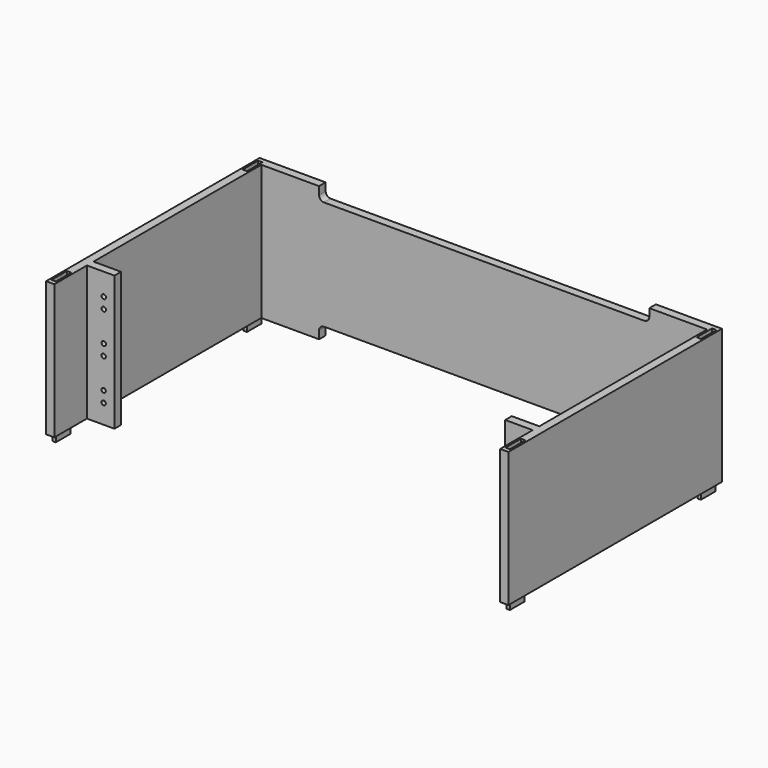
from build123d import *

# Parameters (mm, degrees)
F0_W          = 5
F0_H          = 1.5
F0_W_2        = 0.8
F0_H_2        = 3.5
F0_W_3        = 0.6
F0_H_3        = 3.3
F0_H_4        = 2.7
F0_H_5        = 0.6
F1_DEPTH      = 23
F1_DEPTH_BACK = 1.5
F3_D          = 0.8
F3_DEPTH      = 2
F3_TIP        = 0.2403442476
F5_D          = 0.8
F5_DEPTH      = 2
F5_TIP        = 0.2403442476
F6_DEPTH      = 2.8
F7_START      = 21.5
F7_DEPTH      = 1.5
F9_DEPTH      = 2


# Not quite as in the source:
# - a feature names something its author has since deleted; it is built from what else it names


with BuildPart() as f1:
    # F0 (on Top) → F1 (new body, two sides)
    with BuildSketch(Plane.XY) as f1_sk:
        with Locations((-38.0453250408, -14.9690947816)):
            Rectangle(F0_W, F0_H)
        Polygon((-42.0453250408, -23.1190947816), (-40.5453250408, -23.1190947816), (-40.5453250408, -15.7190947816), (-40.5453250408, -14.2190947816), (-40.5453250408, 23.8809052184), (-40.8953250408, 23.8809052184), (-40.8953250408, 21.0809052184), (-41.6953250408, 21.0809052184), (-41.6953250408, 23.8809052184), (-42.0453250408, 23.8809052184), align=None)
        with Locations((-41.2953250408, -20.5690947816)):
            Rectangle(F0_W_2, F0_H_2, mode=Mode.SUBTRACT)
        Polygon((-42.0453250408, 25.3809052184), (-42.0453250408, 23.8809052184), (-41.6953250408, 23.8809052184), (-41.6953250408, 24.5809052184), (-40.8953250408, 24.5809052184), (-40.8953250408, 23.8809052184), (-40.5453250408, 23.8809052184), (40.4546749592, 23.8809052184), (40.8046749592, 23.8809052184), (40.8046749592, 24.5809052184), (41.6046749592, 24.5809052184), (41.6046749592, 23.8809052184), (41.9546749592, 23.8809052184), (41.9546749592, 25.3809052184), align=None)
        Polygon((40.8046749592, 23.8809052184), (40.4546749592, 23.8809052184), (40.4546749592, -14.2186603174), (40.4546749592, -15.7186603174), (40.4546749592, -23.1190947816), (41.9546749592, -23.1190947816), (41.9546749592, 23.8809052184), (41.6046749592, 23.8809052184), (41.6046749592, 21.0809052184), (40.8046749592, 21.0809052184), align=None)
        with Locations((41.2046749592, -20.5690947816)):
            Rectangle(F0_W_2, F0_H_2, mode=Mode.SUBTRACT)
        with Locations((37.9546749592, -14.9686603174)):
            Rectangle(F0_W, F0_H)
        with Locations((-41.2953250408, -20.5690947816)):
            Rectangle(F0_W_2, F0_H_2)
        with Locations((-41.2953250408, -20.5690947816)):
            Rectangle(F0_W_3, F0_H_3, mode=Mode.SUBTRACT)
        with Locations((41.2046749592, -20.5690947816)):
            Rectangle(F0_W_2, F0_H_2)
        with Locations((41.2046749592, -20.5690947816)):
            Rectangle(F0_W_3, F0_H_3, mode=Mode.SUBTRACT)
        Polygon((40.9046749592, 23.8809052184), (40.8046749592, 23.8809052184), (40.8046749592, 21.0809052184), (41.6046749592, 21.0809052184), (41.6046749592, 23.8809052184), (41.5046749592, 23.8809052184), (41.5046749592, 21.1809052184), (40.9046749592, 21.1809052184), align=None)
        Polygon((40.8046749592, 24.5809052184), (40.8046749592, 23.8809052184), (40.9046749592, 23.8809052184), (40.9046749592, 24.4809052184), (41.5046749592, 24.4809052184), (41.5046749592, 23.8809052184), (41.6046749592, 23.8809052184), (41.6046749592, 24.5809052184), align=None)
        Polygon((-41.6953250408, 24.5809052184), (-41.6953250408, 23.8809052184), (-41.5953250408, 23.8809052184), (-41.5953250408, 24.4809052184), (-40.9953250408, 24.4809052184), (-40.9953250408, 23.8809052184), (-40.8953250408, 23.8809052184), (-40.8953250408, 24.5809052184), align=None)
        Polygon((-41.5953250408, 23.8809052184), (-41.6953250408, 23.8809052184), (-41.6953250408, 21.0809052184), (-40.8953250408, 21.0809052184), (-40.8953250408, 23.8809052184), (-40.9953250408, 23.8809052184), (-40.9953250408, 21.1809052184), (-41.5953250408, 21.1809052184), align=None)
        with Locations((-41.2953250408, -20.5690947816)):
            Rectangle(F0_W_3, F0_H_3)
        with Locations((-41.2953250408, 22.5309052184)):
            Rectangle(F0_W_3, F0_H_4)
        with Locations((41.2046749592, -20.5690947816)):
            Rectangle(F0_W_3, F0_H_3)
        with Locations((41.2046749592, 22.5309052184)):
            Rectangle(F0_W_3, F0_H_4)
        with Locations((41.2046749592, 24.1809052184)):
            Rectangle(F0_W_3, F0_H_5)
        with Locations((-41.2953250408, 24.1809052184)):
            Rectangle(F0_W_3, F0_H_5)
    extrude(amount=F1_DEPTH)
    extrude(f1_sk.sketch, amount=-F1_DEPTH_BACK)

    # F3
    with Locations(Plane.XZ.offset(15.7190947816)):
        with Locations((-37.4758429825, 18.9999998622), (-37.4758429825, 16.9999998622), (-37.4758429825, 11.4999998622), (-37.5126936273, 9.5), (-37.5126936273, 3.9999998622), (-37.5126936273, 2)):
            Hole(F3_D / 2, depth=F3_DEPTH)
            with Locations((0, 0, -(F3_DEPTH + F3_TIP / 2))):  # 118° drill point
                Cone(0, F3_D / 2, F3_TIP, mode=Mode.SUBTRACT)

    # F5
    with Locations(Plane.XZ.offset(15.7186603174)):
        with Locations((37.5221328411, 19.00000019), (37.5221328411, 17.00000019), (37.5221328411, 11.50000019), (37.4725908041, 9.5000003278), (37.4725908041, 4.00000019), (37.4725908041, 2.0000003278)):
            Hole(F5_D / 2, depth=F5_DEPTH)
            with Locations((0, 0, -(F5_DEPTH + F5_TIP / 2))):  # 118° drill point
                Cone(0, F5_D / 2, F5_TIP, mode=Mode.SUBTRACT)

    # F0 (on Top) → F6 (join)
    with BuildSketch(Plane.XY):
        with Locations((-41.2953250408, 22.5309052184)):
            Rectangle(F0_W_3, F0_H_4)
        with Locations((-41.2953250408, 24.1809052184)):
            Rectangle(F0_W_3, F0_H_5)
        with Locations((-41.2953250408, -20.5690947816)):
            Rectangle(F0_W_3, F0_H_3)
        with Locations((41.2046749592, 22.5309052184)):
            Rectangle(F0_W_3, F0_H_4)
        with Locations((41.2046749592, 24.1809052184)):
            Rectangle(F0_W_3, F0_H_5)
        with Locations((41.2046749592, -20.5690947816)):
            Rectangle(F0_W_3, F0_H_3)
    extrude(amount=-F6_DEPTH)

    # F0 (on Top) → F7 (cut)
    with BuildSketch(Plane.XY.offset(F7_START)):
        with Locations((-41.2953250408, -20.5690947816)):
            Rectangle(F0_W_2, F0_H_2)
        with Locations((-41.2953250408, -20.5690947816)):
            Rectangle(F0_W_3, F0_H_3, mode=Mode.SUBTRACT)
        with Locations((41.2046749592, -20.5690947816)):
            Rectangle(F0_W_2, F0_H_2)
        with Locations((41.2046749592, -20.5690947816)):
            Rectangle(F0_W_3, F0_H_3, mode=Mode.SUBTRACT)
        with Locations((-41.2953250408, -20.5690947816)):
            Rectangle(F0_W_3, F0_H_3)
        with Locations((41.2046749592, -20.5690947816)):
            Rectangle(F0_W_3, F0_H_3)
        with Locations((-41.2953250408, 22.5309052184)):
            Rectangle(F0_W_3, F0_H_4)
        with Locations((41.2046749592, 22.5309052184)):
            Rectangle(F0_W_3, F0_H_4)
        Polygon((-41.5953250408, 23.8809052184), (-41.6953250408, 23.8809052184), (-41.6953250408, 21.0809052184), (-40.8953250408, 21.0809052184), (-40.8953250408, 23.8809052184), (-40.9953250408, 23.8809052184), (-40.9953250408, 21.1809052184), (-41.5953250408, 21.1809052184), align=None)
        Polygon((40.9046749592, 23.8809052184), (40.8046749592, 23.8809052184), (40.8046749592, 21.0809052184), (41.6046749592, 21.0809052184), (41.6046749592, 23.8809052184), (41.5046749592, 23.8809052184), (41.5046749592, 21.1809052184), (40.9046749592, 21.1809052184), align=None)
        with Locations((-41.2953250408, 24.1809052184)):
            Rectangle(F0_W_3, F0_H_5)
        with Locations((41.2046749592, 24.1809052184)):
            Rectangle(F0_W_3, F0_H_5)
        Polygon((40.8046749592, 24.5809052184), (40.8046749592, 23.8809052184), (40.9046749592, 23.8809052184), (40.9046749592, 24.4809052184), (41.5046749592, 24.4809052184), (41.5046749592, 23.8809052184), (41.6046749592, 23.8809052184), (41.6046749592, 24.5809052184), align=None)
        Polygon((-41.6953250408, 24.5809052184), (-41.6953250408, 23.8809052184), (-41.5953250408, 23.8809052184), (-41.5953250408, 24.4809052184), (-40.9953250408, 24.4809052184), (-40.9953250408, 23.8809052184), (-40.8953250408, 23.8809052184), (-40.8953250408, 24.5809052184), align=None)
    extrude(amount=F7_DEPTH, mode=Mode.SUBTRACT)

    # F8 (on face) → F9 (cut)
    with BuildSketch(Plane(origin=(0, 25.3809052184, 0), x_dir=(-1, 0, 0), z_dir=(0, 1, 0))):
        with BuildLine():
            ThreePointArc((-29.9546749592, 21.5864117908), (-29.6910710623, 20.9500156878), (-29.0546749592, 20.6864117908))
            Line((-29.0546749592, 20.6864117908), (29.1453250408, 20.6864117908))
            ThreePointArc((29.1453250408, 20.6864117908), (29.7817211439, 20.9500156878), (30.0453250408, 21.5864117908))
            Line((30.0453250408, 21.5864117908), (30.0453250408, 23))
            Line((30.0453250408, 23), (-29.9546749592, 23))
            Line((-29.9546749592, 23), (-29.9546749592, 21.5864117908))
        make_face()
        with BuildLine():
            Line((-29.9546749592, -0.0864118039), (-29.9546749592, -1.500000013))
            Line((-29.9546749592, -1.500000013), (30.0453250408, -1.500000013))
            Line((30.0453250408, -1.500000013), (30.0453250408, -0.0864118039))
            ThreePointArc((30.0453250408, -0.0864118039), (29.7817211439, 0.5499842992), (29.1453250408, 0.8135881961))
            Line((29.1453250408, 0.8135881961), (-29.0546749592, 0.8135881961))
            ThreePointArc((-29.0546749592, 0.8135881961), (-29.6910710623, 0.5499842992), (-29.9546749592, -0.0864118039))
        make_face()
    extrude(amount=-F9_DEPTH, mode=Mode.SUBTRACT)


solid = f1.part
